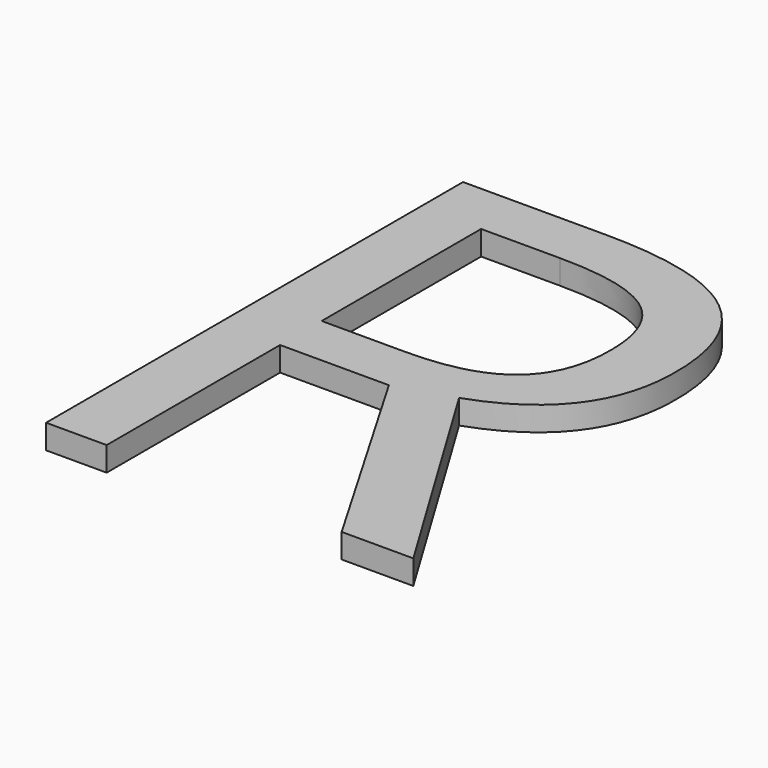
from build123d import *

# Parameters (mm, degrees)
F0_TEXT_SIZE = 120.1313937119
F1_DEPTH     = 4


# Not quite as in the source:
# - Text() gives the source's letters only with a copy of the font that has no kerning and outlines rounded to 1/6400 em; it was checked with that copy


with BuildPart() as f1:
    # F0 (on Top) → F1 (new body)
    with BuildSketch(Plane.XY):
        with Locations((-34.1426085471, -49.2791602925)):
            Text('R', F0_TEXT_SIZE, font='Open Sans', text_align=(TextAlign.LEFT, TextAlign.BOTTOM))
    extrude(amount=F1_DEPTH)


solid = f1.part
